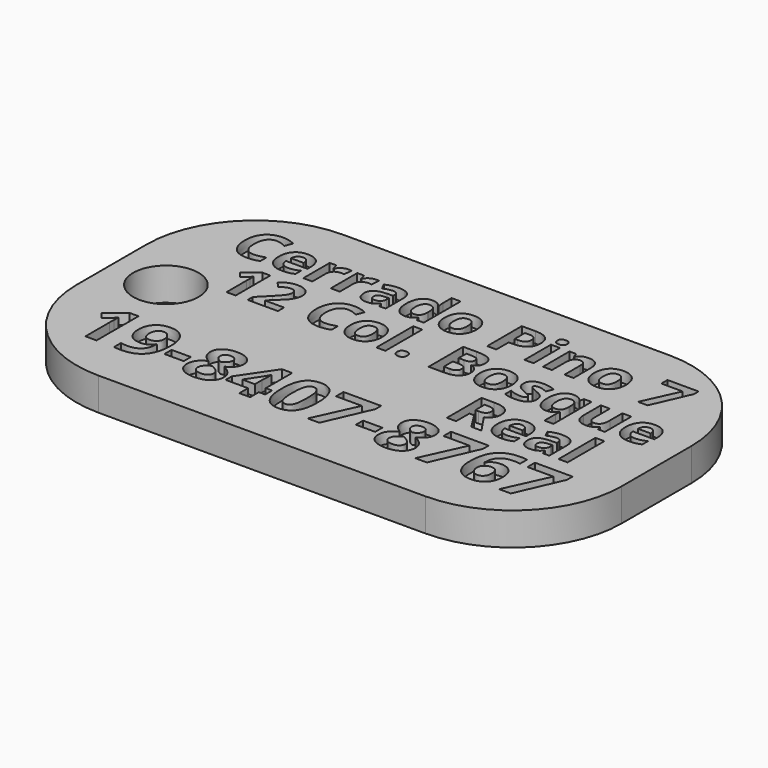
from build123d import *

# Parameters (mm, degrees)
F0_R           = 3
F1_DEPTH       = 3
F2_TEXT_SIZE   = 8.3333333333
F2_TEXT_SIZE_2 = 6.25
F2_TEXT_SIZE_3 = 12.771995777
F3_DEPTH       = 1
F4_TEXT_SIZE   = 5.5555555556
F4_TEXT_SIZE_2 = 6.7407763304
F5_DEPTH       = 1


# Not quite as in the source:
# - Text() gives the source's letters only with a copy of the font that has no kerning and outlines rounded to 1/6400 em; it was checked with that copy


with BuildPart() as f1:
    # F0 (on Top) → F1 (new body)
    with BuildSketch(Plane.XY):
        with BuildLine():
            Line((15, 14), (-15, 14))
            ThreePointArc((-15, 14), (-22.0710678119, 11.0710678119), (-25, 4))
            Line((-25, 4), (-25, -4))
            ThreePointArc((-25, -4), (-22.0710678119, -11.0710678119), (-15, -14))
            Line((-15, -14), (15, -14))
            ThreePointArc((15, -14), (22.0710678119, -11.0710678119), (25, -4))
            Line((25, -4), (25, 4))
            ThreePointArc((25, 4), (22.0710678119, 11.0710678119), (15, 14))
        make_face()
        with Locations((-20, 0)):
            Circle(F0_R, mode=Mode.SUBTRACT)
    extrude(amount=F1_DEPTH)

    # F2 (on face) → F3 (cut)
    with BuildSketch(Plane(origin=(0, 0, 0), x_dir=(1, 0, 0), z_dir=(0, 0, -1))):
        with Locations((-11.5658252372, 6.3531089665)):
            Text('PLAYA', F2_TEXT_SIZE, font='Open Sans', font_style=FontStyle.BOLD, text_align=(TextAlign.LEFT, TextAlign.BOTTOM))
        with Locations((-16.646174714, 0.3959320411)):
            Text('DEL CARMEN', F2_TEXT_SIZE_2, font='Open Sans', font_style=FontStyle.BOLD, text_align=(TextAlign.LEFT, TextAlign.BOTTOM))
        with Locations((-11.70766633, -11.0264895484)):
            Text('2017', F2_TEXT_SIZE_3, font='Open Sans', font_style=FontStyle.BOLD, text_align=(TextAlign.LEFT, TextAlign.BOTTOM))
    extrude(amount=-F3_DEPTH, mode=Mode.SUBTRACT)

    # F4 (on face) → F5 (cut)
    with BuildSketch(Plane.XY.offset(3)):
        with Locations((-20.2249070664, 6.9574497565)):
            Text('Cerrado Pino 7', F4_TEXT_SIZE, font='Open Sans', font_style=FontStyle.BOLD, text_align=(TextAlign.LEFT, TextAlign.BOTTOM))
        with Locations((-17.3645950854, 1.8325453429)):
            Text('12 Col. Bosque', F4_TEXT_SIZE, font='Open Sans', font_style=FontStyle.BOLD, text_align=(TextAlign.LEFT, TextAlign.BOTTOM))
        with Locations((8.0942544155, -3.5316932909)):
            Text('Real', F4_TEXT_SIZE, font='Open Sans', font_style=FontStyle.BOLD, text_align=(TextAlign.LEFT, TextAlign.BOTTOM))
        with Locations((-21.2813373655, -9.8344376311)):
            Text('19-8407-8767', F4_TEXT_SIZE_2, font='Open Sans', font_style=FontStyle.BOLD, text_align=(TextAlign.LEFT, TextAlign.BOTTOM))
    extrude(amount=-F5_DEPTH, mode=Mode.SUBTRACT)


solid = f1.part
